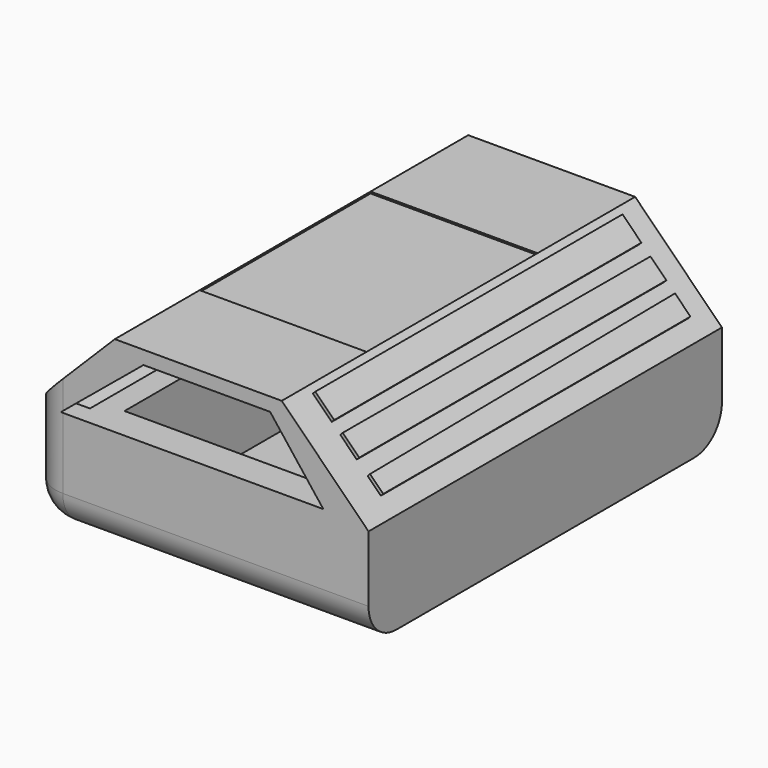
from build123d import *

# Parameters (mm, degrees)
F0_W         = 19.62069033
F0_H         = 25.4568966
F1_DEPTH     = 5.4
F2_SIZE      = 5
F3_SIZE      = 5
F4_W         = 22.1276450902
F4_H         = 1.5373004135
F5_DEPTH     = 0.2
F7_DEPTH     = 25.5
F8_W         = 23.348543793
F8_H         = 5.9792976826
F9_DEPTH     = 1.7
F10_R        = 2
F11_T1_DEPTH = 28.4568966
F11_T3_DEPTH = 8.8
F11_T6_ANGLE = 90
F12_T1_DEPTH = 22.62069033
F12_T3_DEPTH = 8.8
F12_T6_ANGLE = 90.0000000053
F14_DEPTH    = 5.6
F15_W        = 9.62069033
F15_H        = 12.3144993559
F16_DEPTH    = 0.1


# Not quite as in the source:
# - a fillet or chamfer that OpenCascade refuses, or shapes differently, is made with other operations: its cross-section is extruded or revolved along the edge and cut away or added


with BuildPart() as f1:
    # F0 (on Top) → F1 (new body, symmetric)
    with BuildSketch(Plane.XY):
        Rectangle(F0_W, F0_H)
    extrude(amount=F1_DEPTH, both=True)

    # F2
    f2_edges = [f1.edges().sort_by_distance(p)[0] for p in [
        (-9.810345, 0, 5.4),
    ]]
    chamfer(f2_edges, length=F2_SIZE)

    # F3
    f3_edges = [f1.edges().sort_by_distance(p)[0] for p in [
        (9.810345, 0, 5.4),
    ]]
    chamfer(f3_edges, length=F3_SIZE)

    # F4 (on face) → F5 (join)
    with BuildSketch(Plane(origin=(5.1051725825, 0, 5.1051725825), x_dir=(0, 1, 0), z_dir=(0.7071067812, 0, 0.7071067812))):
        with Locations((0.2083815634, -0.7686502067)):
            Rectangle(F4_W, F4_H)
        Polygon((11.2722041085, -2.2796541452), (-10.8554409817, -2.2294183727), (-10.8554409817, -3.5751299001), (11.2722041085, -3.5751299001), align=None)
        Polygon((11.2722041085, -4.2798109353), (-10.8554409817, -4.4601280242), (-10.8554409817, -5.5370246992), (11.2722041085, -5.5370246992), align=None)
    extrude(amount=F5_DEPTH)

    # F6 (on face) → F7 (cut)
    with BuildSketch(Plane.XZ.offset(12.7284483)):
        Polygon((4.140063189, 4.6230903827), (-3.1588820275, 4.6230903827), (-7.9239970073, 0.6864351453), (7.2048916481, 0.6864351453), align=None)
    extrude(amount=-F7_DEPTH, mode=Mode.SUBTRACT)

    # F8 (on face) → F9 (cut)
    with BuildSketch(Plane(origin=(-5.1051725825, 0, 5.1051725825), x_dir=(0, -1, 0), z_dir=(-0.7071067812, 0, 0.7071067812))):
        with Locations((-0.0411020592, -2.9896488413)):
            Rectangle(F8_W, F8_H)
    extrude(amount=-F9_DEPTH, mode=Mode.SUBTRACT)

    # F10
    f10_edges = [f1.edges().sort_by_distance(p)[0] for p in [
        (0, -12.728448, -5.4),
    ]]
    fillet(f10_edges, radius=F10_R)

    # F11: fillet of radius 2 on 1 edges, made by hand

    # F11_s2 → F11_t1 (cut)
    with BuildSketch(Plane.XZ.offset(-17.7284483)):
        with BuildLine():
            ThreePointArc((-7.810345165, -5.4), (-9.2245587274, -4.8142135624), (-9.810345165, -3.4))
            Line((-9.810345165, -3.4), (-9.810345165, -5.4))
            Line((-9.810345165, -5.4), (-7.810345165, -5.4))
        make_face()
    extrude(amount=F11_T1_DEPTH, mode=Mode.SUBTRACT)

    # F11_s4 → F11_t3 (cut)
    with BuildSketch(Plane.XY.offset(-3.4)):
        with BuildLine():
            ThreePointArc((-7.810345165, -12.7284483), (-9.2245587274, -12.1426618624), (-9.810345165, -10.7284483))
            Line((-9.810345165, -10.7284483), (-9.810345165, -12.7284483))
            Line((-9.810345165, -12.7284483), (-7.810345165, -12.7284483))
        make_face()
    extrude(amount=F11_T3_DEPTH, mode=Mode.SUBTRACT)

    # F11_s5 → F11_t6 (revolve, cut)
    with BuildSketch(Plane.XZ.offset(10.7284483)):
        with BuildLine():
            ThreePointArc((-7.810345165, -5.4), (-9.2245587274, -4.8142135624), (-9.810345165, -3.4))
            Line((-9.810345165, -3.4), (-9.810345165, -5.4))
            Line((-9.810345165, -5.4), (-7.810345165, -5.4))
        make_face()
    revolve(axis=Axis((-9.810345165, -10.7284483, -3.4), (-1, 0, 0)), revolution_arc=F11_T6_ANGLE, mode=Mode.SUBTRACT)

    # F12: fillet of radius 2 on 1 edges, made by hand

    # F12_s2 → F12_t1 (cut)
    with BuildSketch(Plane.YZ.offset(-7.810345165)):
        with BuildLine():
            ThreePointArc((10.7284483, -5.4), (12.1426618624, -4.8142135624), (12.7284483, -3.4))
            Line((12.7284483, -3.4), (12.7284483, -5.4))
            Line((12.7284483, -5.4), (10.7284483, -5.4))
        make_face()
    extrude(amount=F12_T1_DEPTH, mode=Mode.SUBTRACT)

    # F12_s4 → F12_t3 (cut)
    with BuildSketch(Plane.XY.offset(-3.4)):
        with BuildLine():
            ThreePointArc((-7.810345165, 12.7284483), (-9.2245587274, 12.1426618624), (-9.810345165, 10.7284483))
            Line((-9.810345165, 10.7284483), (-9.810345165, 12.7284483))
            Line((-9.810345165, 12.7284483), (-7.810345165, 12.7284483))
        make_face()
    extrude(amount=F12_T3_DEPTH, mode=Mode.SUBTRACT)

    # F12_s5 → F12_t6 (revolve, cut)
    with BuildSketch(Plane.YZ.offset(-7.8103451651)):
        with BuildLine():
            ThreePointArc((12.7284483, -3.4), (12.1426618624, -4.8142135624), (10.7284483, -5.4))
            Line((10.7284483, -5.4), (12.7284483, -5.4))
            Line((12.7284483, -5.4), (12.7284483, -3.4))
        make_face()
    revolve(axis=Axis((-7.8103451651, 12.7284483, -3.4000000001), (0, 1, 0)), revolution_arc=F12_T6_ANGLE, mode=Mode.SUBTRACT)

    # F13 (on face) → F14 (cut)
    with BuildSketch(Plane.XY.offset(0.6864351453)):
        Polygon((6.1108670197, -10.853772983), (6.3247303478, 11.9756069034), (-5.7491413318, 11.2674161792), (-5.7491413318, -10.853772983), align=None)
    extrude(amount=-F14_DEPTH, mode=Mode.SUBTRACT)

    # F15 (on face) → F16 (cut)
    with BuildSketch(Plane.XY.offset(5.4)):
        with Locations((0, -0.4627322778)):
            Rectangle(F15_W, F15_H)
    extrude(amount=-F16_DEPTH, mode=Mode.SUBTRACT)


solid = f1.part
